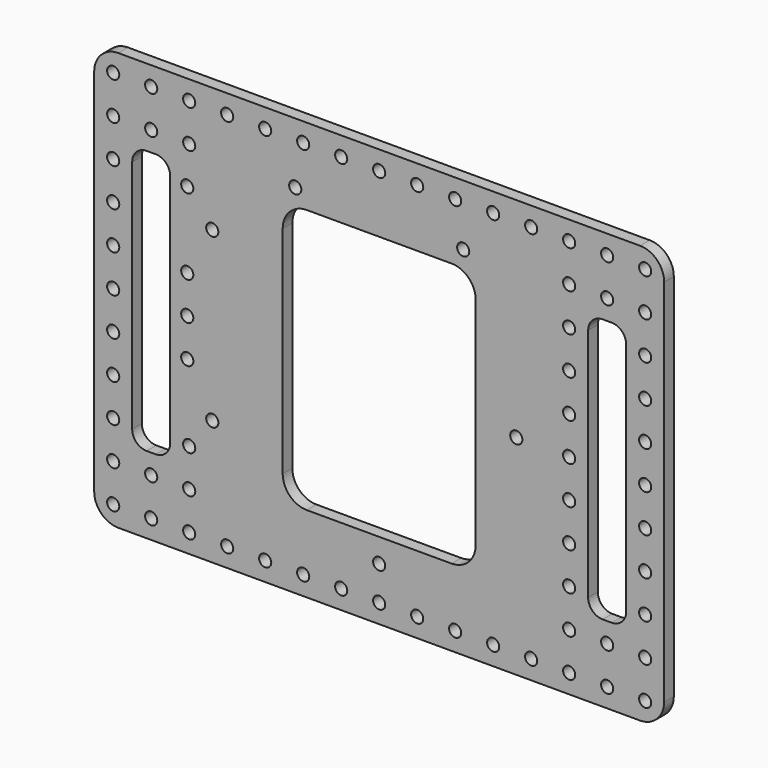
from build123d import *

# Parameters (mm, degrees)
F0_R     = 1.6
F1_DEPTH = 3.175


# Not quite as in the source:
# - a length typed as a fraction of an inch, garbled in the dataset ("3 / 203.2 mm" for 3/8 in), is restored


with BuildPart() as f1:
    # F0 (on Front) → F1 (new body)
    with BuildSketch(Plane.XZ):
        with BuildLine():
            Line((143.65, 0), (6.35, 0))
            ThreePointArc((6.35, 0), (1.8598719395, -1.8598719395), (0, -6.35))
            Line((0, -6.35), (0, -103.65))
            ThreePointArc((0, -103.65), (1.8598719395, -108.1401280605), (6.35, -110))
            Line((6.35, -110), (143.65, -110))
            ThreePointArc((143.65, -110), (148.1401280605, -108.1401280605), (150, -103.65))
            Line((150, -103.65), (150, -6.35))
            ThreePointArc((150, -6.35), (148.1401280605, -1.8598719395), (143.65, 0))
        make_face()
        with Locations((5, -105)):
            Circle(F0_R, mode=Mode.SUBTRACT)
        with Locations((15, -105)):
            Circle(F0_R, mode=Mode.SUBTRACT)
        with Locations((25, -105)):
            Circle(F0_R, mode=Mode.SUBTRACT)
        with Locations((35, -105)):
            Circle(F0_R, mode=Mode.SUBTRACT)
        with Locations((5, -95)):
            Circle(F0_R, mode=Mode.SUBTRACT)
        with Locations((15, -95)):
            Circle(F0_R, mode=Mode.SUBTRACT)
        with Locations((5, -85)):
            Circle(F0_R, mode=Mode.SUBTRACT)
        with Locations((25, -95)):
            Circle(F0_R, mode=Mode.SUBTRACT)
        with Locations((25, -85)):
            Circle(F0_R, mode=Mode.SUBTRACT)
        with Locations((45, -105)):
            Circle(F0_R, mode=Mode.SUBTRACT)
        with Locations((55, -105)):
            Circle(F0_R, mode=Mode.SUBTRACT)
        with Locations((65, -105)):
            Circle(F0_R, mode=Mode.SUBTRACT)
        with Locations((5, -75)):
            Circle(F0_R, mode=Mode.SUBTRACT)
        with Locations((31.077, -77.1057)):
            Circle(F0_R, mode=Mode.SUBTRACT)
        with Locations((5, -65)):
            Circle(F0_R, mode=Mode.SUBTRACT)
        with BuildLine():
            ThreePointArc((10, -24.0538), (11.1159231637, -21.3597231637), (13.81, -20.2438))
            Line((13.81, -20.2438), (16.19, -20.2438))
            ThreePointArc((16.19, -20.2438), (18.8840768363, -21.3597231637), (20, -24.0538))
            Line((20, -24.0538), (20, -85.9536))
            ThreePointArc((20, -85.9536), (18.8840768363, -88.6476768363), (16.19, -89.7636))
            Line((16.19, -89.7636), (13.81, -89.7636))
            ThreePointArc((13.81, -89.7636), (11.1159231637, -88.6476768363), (10, -85.9536))
            Line((10, -85.9536), (10, -24.0538))
        make_face(mode=Mode.SUBTRACT)
        with Locations((24.492, -65)):
            Circle(F0_R, mode=Mode.SUBTRACT)
        with Locations((75, -105)):
            Circle(F0_R, mode=Mode.SUBTRACT)
        with Locations((85, -105)):
            Circle(F0_R, mode=Mode.SUBTRACT)
        with Locations((95, -105)):
            Circle(F0_R, mode=Mode.SUBTRACT)
        with Locations((105, -105)):
            Circle(F0_R, mode=Mode.SUBTRACT)
        with Locations((75, -95.9955)):
            Circle(F0_R, mode=Mode.SUBTRACT)
        with Locations((115, -105)):
            Circle(F0_R, mode=Mode.SUBTRACT)
        with Locations((125, -105)):
            Circle(F0_R, mode=Mode.SUBTRACT)
        with Locations((135, -105)):
            Circle(F0_R, mode=Mode.SUBTRACT)
        with Locations((145, -105)):
            Circle(F0_R, mode=Mode.SUBTRACT)
        with Locations((125, -95)):
            Circle(F0_R, mode=Mode.SUBTRACT)
        with Locations((125, -85)):
            Circle(F0_R, mode=Mode.SUBTRACT)
        with Locations((135, -95)):
            Circle(F0_R, mode=Mode.SUBTRACT)
        with Locations((145, -95)):
            Circle(F0_R, mode=Mode.SUBTRACT)
        with Locations((145, -85)):
            Circle(F0_R, mode=Mode.SUBTRACT)
        with BuildLine():
            Line((49.6062, -83.4136), (49.6062, -26.5938))
            ThreePointArc((49.6062, -26.5938), (51.4660719395, -22.1036719395), (55.9562, -20.2438))
            Line((55.9562, -20.2438), (94.0562, -20.2438))
            ThreePointArc((94.0562, -20.2438), (98.5463280605, -22.1036719395), (100.4062, -26.5938))
            Line((100.4062, -26.5938), (100.4062, -83.4136))
            ThreePointArc((100.4062, -83.4136), (98.5463280605, -87.9037280605), (94.0562, -89.7636))
            Line((94.0562, -89.7636), (55.9562, -89.7636))
            ThreePointArc((55.9562, -89.7636), (51.4660719395, -87.9037280605), (49.6062, -83.4136))
        make_face(mode=Mode.SUBTRACT)
        with Locations((111.077, -55.0037)):
            Circle(F0_R, mode=Mode.SUBTRACT)
        with Locations((125, -75)):
            Circle(F0_R, mode=Mode.SUBTRACT)
        with Locations((145, -75)):
            Circle(F0_R, mode=Mode.SUBTRACT)
        with Locations((125, -65)):
            Circle(F0_R, mode=Mode.SUBTRACT)
        with Locations((145, -65)):
            Circle(F0_R, mode=Mode.SUBTRACT)
        with BuildLine():
            ThreePointArc((130, -24.0538), (131.1159231637, -21.3597231637), (133.81, -20.2438))
            Line((133.81, -20.2438), (136.19, -20.2438))
            ThreePointArc((136.19, -20.2438), (138.8840768363, -21.3597231637), (140, -24.0538))
            Line((140, -24.0538), (140, -85.9536))
            ThreePointArc((140, -85.9536), (138.8840768363, -88.6476768363), (136.19, -89.7636))
            Line((136.19, -89.7636), (133.81, -89.7636))
            ThreePointArc((133.81, -89.7636), (131.1159231637, -88.6476768363), (130, -85.9536))
            Line((130, -85.9536), (130, -24.0538))
        make_face(mode=Mode.SUBTRACT)
        with Locations((5, -55)):
            Circle(F0_R, mode=Mode.SUBTRACT)
        with Locations((5, -45)):
            Circle(F0_R, mode=Mode.SUBTRACT)
        with Locations((24.492, -55)):
            Circle(F0_R, mode=Mode.SUBTRACT)
        with Locations((24.492, -45)):
            Circle(F0_R, mode=Mode.SUBTRACT)
        with Locations((5, -35)):
            Circle(F0_R, mode=Mode.SUBTRACT)
        with Locations((31.077, -32.9057)):
            Circle(F0_R, mode=Mode.SUBTRACT)
        with Locations((5, -25)):
            Circle(F0_R, mode=Mode.SUBTRACT)
        with Locations((5, -15)):
            Circle(F0_R, mode=Mode.SUBTRACT)
        with Locations((15, -15)):
            Circle(F0_R, mode=Mode.SUBTRACT)
        with Locations((24.492, -25)):
            Circle(F0_R, mode=Mode.SUBTRACT)
        with Locations((25, -15)):
            Circle(F0_R, mode=Mode.SUBTRACT)
        with Locations((5, -5)):
            Circle(F0_R, mode=Mode.SUBTRACT)
        with Locations((15, -5)):
            Circle(F0_R, mode=Mode.SUBTRACT)
        with Locations((25, -5)):
            Circle(F0_R, mode=Mode.SUBTRACT)
        with Locations((35, -5)):
            Circle(F0_R, mode=Mode.SUBTRACT)
        with Locations((52.9082, -15.9955)):
            Circle(F0_R, mode=Mode.SUBTRACT)
        with Locations((45, -5)):
            Circle(F0_R, mode=Mode.SUBTRACT)
        with Locations((55, -5)):
            Circle(F0_R, mode=Mode.SUBTRACT)
        with Locations((65, -5)):
            Circle(F0_R, mode=Mode.SUBTRACT)
        with Locations((125, -55)):
            Circle(F0_R, mode=Mode.SUBTRACT)
        with Locations((125, -45)):
            Circle(F0_R, mode=Mode.SUBTRACT)
        with Locations((145, -55)):
            Circle(F0_R, mode=Mode.SUBTRACT)
        with Locations((145, -45)):
            Circle(F0_R, mode=Mode.SUBTRACT)
        with Locations((125, -35)):
            Circle(F0_R, mode=Mode.SUBTRACT)
        with Locations((145, -35)):
            Circle(F0_R, mode=Mode.SUBTRACT)
        with Locations((97.1082, -15.9955)):
            Circle(F0_R, mode=Mode.SUBTRACT)
        with Locations((75, -5)):
            Circle(F0_R, mode=Mode.SUBTRACT)
        with Locations((85, -5)):
            Circle(F0_R, mode=Mode.SUBTRACT)
        with Locations((95, -5)):
            Circle(F0_R, mode=Mode.SUBTRACT)
        with Locations((105, -5)):
            Circle(F0_R, mode=Mode.SUBTRACT)
        with Locations((125, -25)):
            Circle(F0_R, mode=Mode.SUBTRACT)
        with Locations((125, -15)):
            Circle(F0_R, mode=Mode.SUBTRACT)
        with Locations((145, -25)):
            Circle(F0_R, mode=Mode.SUBTRACT)
        with Locations((135, -15)):
            Circle(F0_R, mode=Mode.SUBTRACT)
        with Locations((145, -15)):
            Circle(F0_R, mode=Mode.SUBTRACT)
        with Locations((115, -5)):
            Circle(F0_R, mode=Mode.SUBTRACT)
        with Locations((125, -5)):
            Circle(F0_R, mode=Mode.SUBTRACT)
        with Locations((135, -5)):
            Circle(F0_R, mode=Mode.SUBTRACT)
        with Locations((145, -5)):
            Circle(F0_R, mode=Mode.SUBTRACT)
    extrude(amount=F1_DEPTH)


solid = f1.part
